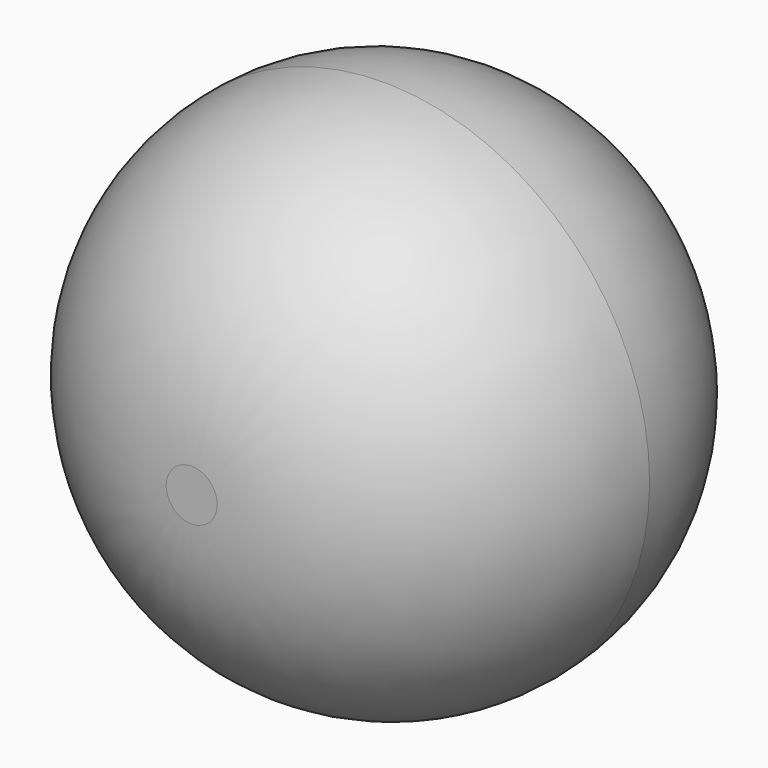
from build123d import *

# Parameters (mm, degrees)
F0_R     = 42.1386103745
F1_DEPTH = 76.2
F2_R     = 38.1
F3_R     = 38.09999


# Not quite as in the source:
# - a fillet or chamfer is up to 0.001 mm smaller than in the source, because OpenCascade refuses the exact size


with BuildPart() as f1:
    # F0 (on Front) → F1 (new body)
    with BuildSketch(Plane.XZ):
        Circle(F0_R)
    extrude(amount=F1_DEPTH)

    # F2
    f2_edges = [f1.edges().sort_by_distance(p)[0] for p in [
        (-42.13861, -76.2, 0),
    ]]
    fillet(f2_edges, radius=F2_R)

    # F3 (radius 38.1 in the source; OpenCascade refuses exactly that, so slightly less here)
    f3_edges = [f1.edges().sort_by_distance(p)[0] for p in [
        (42.13861, -19.05, 0),
        (-42.13861, -38.1, 0),
        (-42.13861, 0, 0),
    ]]
    fillet(f3_edges, radius=F3_R)


solid = f1.part
